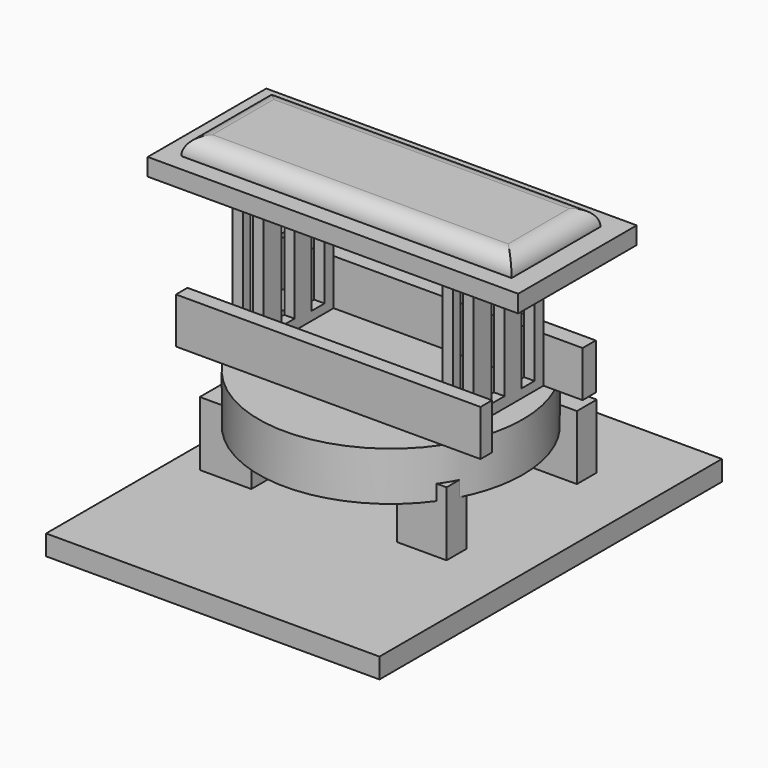
from build123d import *

# Parameters (mm, degrees)
F0_W      = 95.9210544825
F0_H      = 123.1578961015
F1_DEPTH  = 5.8
F2_W      = 14.211
F2_H      = 7.14
F2_W_2    = 14.82887734
F2_H_2    = 7.4144396418
F3_DEPTH  = 18.5
F5_R      = 38.0021383108
F6_DEPTH  = 14
F8_DEPTH  = 13.2
F9_W      = 2.9605254531
F9_H      = 32.5657902285
F10_DEPTH = 40
F12_W     = 106.5789507702
F12_H     = 42.6315842196
F13_DEPTH = 5
F15_W     = 95.0329005718
F15_H     = 31.9736870006
F16_DEPTH = 5
F17_R     = 4.99999
F18_W     = 4.7368425876
F18_H     = 34.638158977
F19_DEPTH = 69.8
F20_W     = 4.737
F20_H     = 34.638
F21_DEPTH = 93.3
F22_W     = 4.737
F22_H     = 34.638
F23_DEPTH = 98.3


# Not quite as in the source:
# - a fillet or chamfer is up to 0.001 mm smaller than in the source, because OpenCascade refuses the exact size


with BuildPart() as f1:
    # F0 (on Top) → F1 (new body)
    with BuildSketch(Plane.XY):
        Rectangle(F0_W, F0_H)
    extrude(amount=F1_DEPTH)

    # F2 (on face) → F3 (join)
    with BuildSketch(Plane.XY.offset(5.8)):
        with Locations((-33.1652933639, 33.6907944659)):
            Rectangle(F2_W, F2_H)
        with Locations((23.060855536, 35.2354664353)):
            Rectangle(F2_W, F2_H)
        with Locations((23.3697903186, -12.0315703675)):
            Rectangle(F2_W, F2_H)
        with Locations((-32.8563585813, -12.2032872729)):
            Rectangle(F2_W_2, F2_H_2)
    extrude(amount=F3_DEPTH)

    # F5 (on offset) → F6 (join)
    with BuildSketch(Plane.XY.offset(19.9)):
        with Locations((-3.2565793954, 6.5131578594)):
            Circle(F5_R)
    extrude(amount=F6_DEPTH)

    # F7 (on face) → F8 (join)
    with BuildSketch(Plane.XY.offset(33.9)):
        with BuildLine():
            Line((30.7933383724, -10.3618418798), (-37.3064971632, -10.3618418798))
            ThreePointArc((-37.3064971632, -10.3618418798), (-36.1766552365, -12.4718657857), (-34.9162250459, -14.5065793768))
            Line((-34.9162250459, -14.5065793768), (28.4030662551, -14.5065793768))
            ThreePointArc((28.4030662551, -14.5065793768), (29.6634964457, -12.4718657857), (30.7933383724, -10.3618418798))
        make_face()
        with BuildLine():
            Line((39.3750034273, -10.3618418798), (30.7933383724, -10.3618418798))
            ThreePointArc((30.7933383724, -10.3618418798), (29.6634964457, -12.4718657857), (28.4030662551, -14.5065793768))
            Line((28.4030662551, -14.5065793768), (39.3750034273, -14.5065793768))
            Line((39.3750034273, -14.5065793768), (39.3750034273, -10.3618418798))
        make_face()
        with BuildLine():
            ThreePointArc((-34.9162250459, -14.5065793768), (-36.1766552365, -12.4718657857), (-37.3064971632, -10.3618418798))
            Line((-37.3064971632, -10.3618418798), (-48.2565825805, -10.3618418798))
            Line((-48.2565825805, -10.3618418798), (-48.2565825805, -14.5065793768))
            Line((-48.2565825805, -14.5065793768), (-34.9162250459, -14.5065793768))
        make_face()
        with BuildLine():
            Line((-37.8681614166, 22.2039483488), (31.3550026259, 22.2039483488))
            ThreePointArc((31.3550026259, 22.2039483488), (30.1557002498, 24.6179109675), (28.7883016181, 26.9407890737))
            Line((28.7883016181, 26.9407890737), (-35.3014604088, 26.9407890737))
            ThreePointArc((-35.3014604088, 26.9407890737), (-36.6688590406, 24.6179109675), (-37.8681614166, 22.2039483488))
        make_face()
        with BuildLine():
            Line((-48.2565825805, 22.2039483488), (-37.8681614166, 22.2039483488))
            ThreePointArc((-37.8681614166, 22.2039483488), (-36.6688590406, 24.6179109675), (-35.3014604088, 26.9407890737))
            Line((-35.3014604088, 26.9407890737), (-48.2565825805, 26.9407890737))
            Line((-48.2565825805, 26.9407890737), (-48.2565825805, 22.2039483488))
        make_face()
        with BuildLine():
            Line((31.3550026259, 22.2039483488), (39.3750034273, 22.2039483488))
            Line((39.3750034273, 22.2039483488), (39.3750034273, 26.9407890737))
            Line((39.3750034273, 26.9407890737), (28.7883016181, 26.9407890737))
            ThreePointArc((28.7883016181, 26.9407890737), (30.1557002498, 24.6179109675), (31.3550026259, 22.2039483488))
        make_face()
    extrude(amount=F8_DEPTH)

    # F9 (on face) → F10 (join)
    with BuildSketch(Plane.XY.offset(33.9)):
        with Locations((-33.7500013411, 5.9210532345)):
            Rectangle(F9_W, F9_H)
        with Locations((26.6447365284, 5.9210532345)):
            Rectangle(F9_W, F9_H)
    extrude(amount=F10_DEPTH)

    # F12 (on offset) → F13 (join)
    with BuildSketch(Plane.XY.offset(73.9)):
        with Locations((-3.5526319407, 7.401315961)):
            Rectangle(F12_W, F12_H)
    extrude(amount=F13_DEPTH)

    # F15 (on face) → F16 (join)
    with BuildSketch(Plane.XY.offset(78.9)):
        with Locations((-3.700658679, 7.105264347)):
            Rectangle(F15_W, F15_H)
    extrude(amount=F16_DEPTH)

    # F17 (radius 5 in the source; OpenCascade refuses exactly that, so slightly less here)
    f17_edges = [f1.edges().sort_by_distance(p)[0] for p in [
        (-3.700659, 23.092108, 83.9),
        (-51.217109, 7.105264, 83.9),
        (-3.700659, -8.881579, 83.9),
        (43.815792, 7.105264, 83.9),
    ]]
    fillet(f17_edges, radius=F17_R)

    # F18 (on face) → F19 (cut)
    with BuildSketch(Plane(origin=(-35.2302640676, 0, 0), x_dir=(0, -1, 0), z_dir=(-1, 0, 0))):
        with Locations((-16.5789490566, 53.742762655)):
            Rectangle(F18_W, F18_H)
    extrude(amount=-F19_DEPTH, mode=Mode.SUBTRACT)

    # F20 (on face) → F21 (cut)
    with BuildSketch(Plane(origin=(-35.2302640676, 0, 0), x_dir=(0, -1, 0), z_dir=(-1, 0, 0))):
        with Locations((-5.8019411517, 54.2707815458)):
            Rectangle(F20_W, F20_H)
    extrude(amount=-F21_DEPTH, mode=Mode.SUBTRACT)

    # F22 (on face) → F23 (cut)
    with BuildSketch(Plane(origin=(-35.2302640676, 0, 0), x_dir=(0, -1, 0), z_dir=(-1, 0, 0))):
        with Locations((5.355990259, 53.9595156418)):
            Rectangle(F22_W, F22_H)
    extrude(amount=-F23_DEPTH, mode=Mode.SUBTRACT)


solid = f1.part
